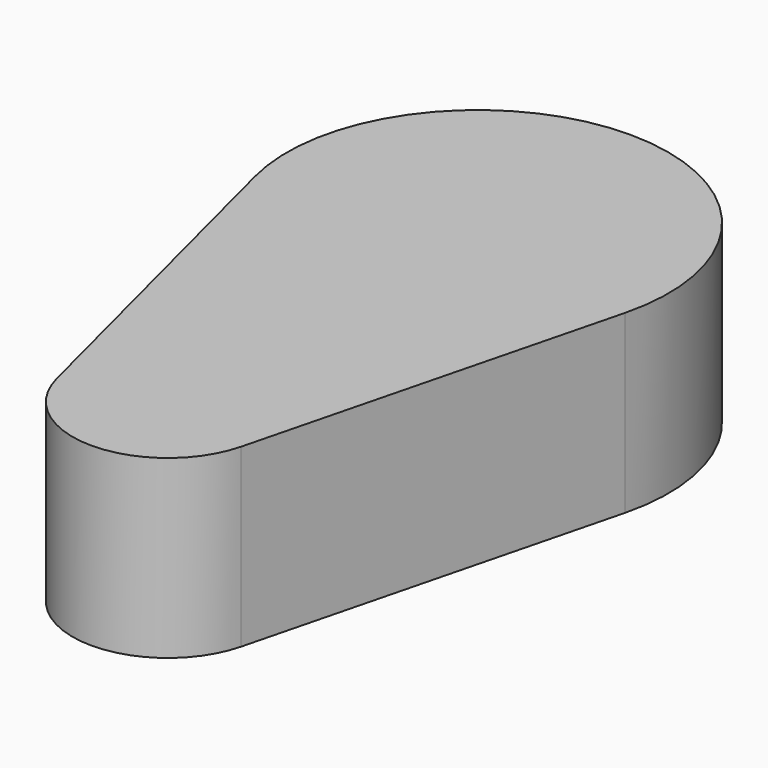
from build123d import *

# Parameters (mm, degrees)
F1_DEPTH = 12.7


# Not quite as in the source:
# - a feature names something its author has since deleted; it is built from what else it names


with BuildPart() as f1:
    # F0 (on Top) → F1 (new body, symmetric)
    with BuildSketch(Plane.XY):
        with BuildLine():
            Line((-26.6787280744, -6.7988147188), (-13.3024417869, -59.2877145153))
            ThreePointArc((-13.3024417869, -59.2877145153), (0, -69.6253179893), (13.3024417869, -59.2877145153))
            Line((13.3024417869, -59.2877145153), (26.6787280744, -6.7988147188))
            ThreePointArc((26.6787280744, -6.7988147188), (0, 27.53140776), (-26.6787280744, -6.7988147188))
        make_face()
    extrude(amount=F1_DEPTH, both=True)


solid = f1.part
